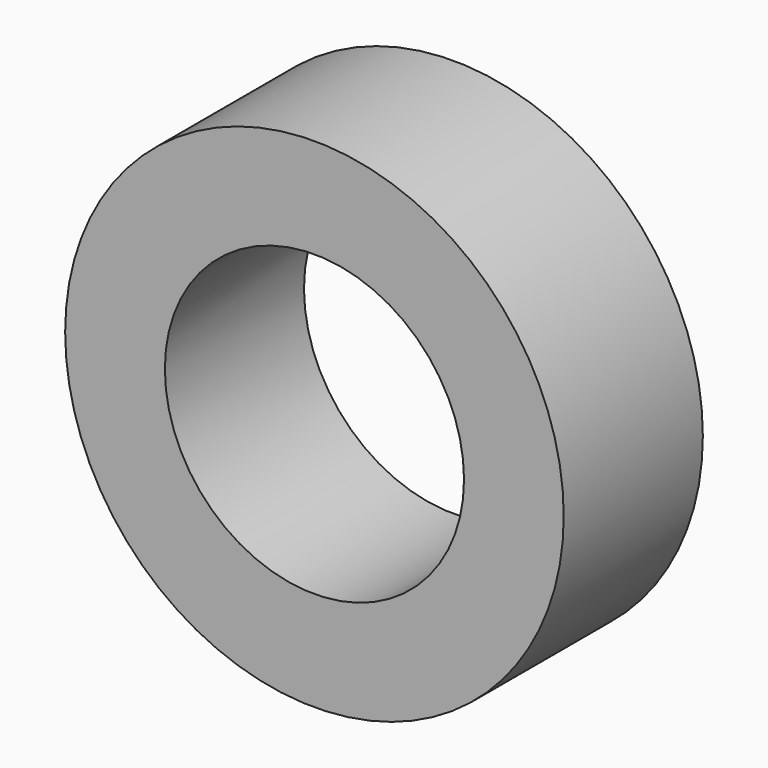
from build123d import *

# Parameters (mm, degrees)
F0_R          = 3.96875
F1_DEPTH      = 2.7686
F2_R          = 2.38125
F3_DEPTH      = 25.4
F3_DEPTH_BACK = 13


# Not quite as in the source:
# - an extrude ends at something that could not be found from the text; its depth is read off the source's solid


with BuildPart() as f1:
    # F0 (on Front) → F1 (new body)
    with BuildSketch(Plane.XZ):
        Circle(F0_R)
    extrude(amount=F1_DEPTH)

    # F2 (on face) → F3 (cut, two sides)
    with BuildSketch(Plane.XZ.offset(2.7686)) as f3_sk:
        Circle(F2_R)
    extrude(amount=-F3_DEPTH, mode=Mode.SUBTRACT)
    extrude(f3_sk.sketch, amount=F3_DEPTH_BACK, mode=Mode.SUBTRACT)


solid = f1.part
